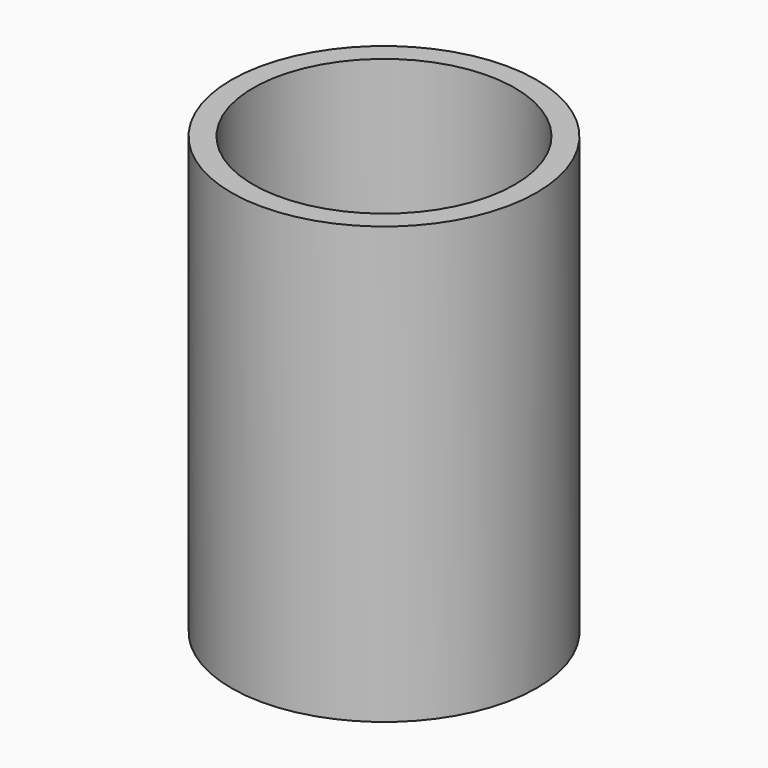
from build123d import *

# Parameters (mm, degrees)
F0_R            = 44.45
F0_R_2          = 38.1
F1_DEPTH        = 127
F2_W            = 6.35
F2_H            = 5.1593752402
F3_DEPTH        = 10.16
F3_COPIES_COUNT = 3


# Not quite as in the source:
# - a pattern or mirror of a feature is missing from the dataset's text; its kind, count and spacing are read off the source's solid


with BuildPart() as f1:
    # F0 (on Top) → F1 (new body)
    with BuildSketch(Plane.XY):
        Circle(F0_R)
        Circle(F0_R_2, mode=Mode.SUBTRACT)
    extrude(amount=F1_DEPTH)

    # F2 (on Top) → F3 (join)
    with BuildSketch(Plane.XY):
        with Locations((-34.925, 0)):
            Rectangle(F2_W, F2_H)
    f3 = extrude(amount=F3_DEPTH)

    # F3_copies: F3 ×3 about axis
    f3_copies_axis = Axis((0, 0, 0), (0, 0, 1))
    for i in range(1, F3_COPIES_COUNT):
        add(f3.rotate(f3_copies_axis, i * 360 / F3_COPIES_COUNT))


solid = f1.part
